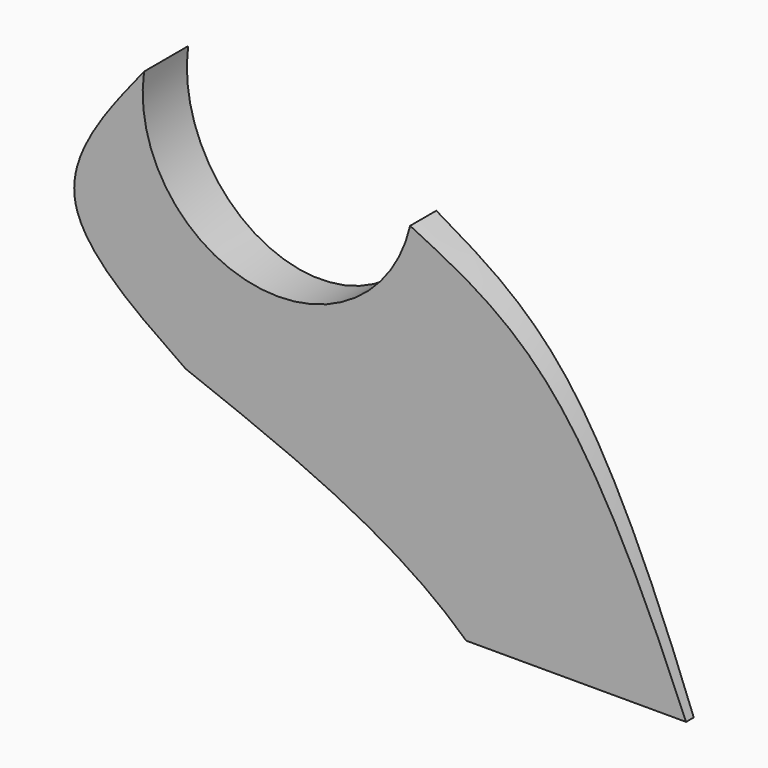
from build123d import *

# Parameters (mm, degrees)
F2_DEPTH = 25.7279276848
F3_DEPTH = 102.7941810931


# Not quite as in the source:
# - a feature names something its author has since deleted; it is built from what else it names


with BuildPart() as f2:
    # F0 (on Front) → F2 (new body, through all)
    with BuildSketch(Plane.XZ):
        with BuildLine():
            ThreePointArc((7.538071066, 90.012077608), (-33.0999025849, 63.2971569556), (-61.4758778659, 102.7931809931))
            add(Edge.make_bspline(
                [(-50.6802275777, 38.4073108435), (-64.2301253741, 47.6853026647), (-91.0055411856, 66.0246371681), (-71.2591028819, 90.6346541889), (-61.4758778659, 102.7931809931)],
                knots=[0, 0, 0, 0, 0.5057307672, 1, 1, 1, 1], degree=3))
            add(Edge.make_bspline(
                [(62.097594142, -64.207687974), (51.1832226367, -40.5716055165), (28.887804967, 7.7111846278), (-23.7900094582, 28.033475615), (-50.6802275777, 38.4073108435)],
                knots=[0, 0, 0, 0, 0.4895343419, 1, 1, 1, 1], degree=3))
            Line((62.097594142, -64.207687974), (96.4130014181, -43.6846762896))
            add(Edge.make_bspline(
                [(96.4130014181, -43.6846762896), (79.9973481318, -1.0988161117), (53.4561883249, 67.712624491), (20.2239489646, 83.857797394), (7.538071066, 90.012077608)],
                knots=[0, 0, 0, 0, 0.6187491541, 1, 1, 1, 1], degree=3))
        make_face()
    extrude(amount=F2_DEPTH)


with BuildPart() as f3:
    # F1 (on Top) → F3 (new body, through all)
    with BuildSketch(Plane.XY):
        Polygon((108.6692065001, -25.7279276848), (-108.6692065001, -7.4702873826), (-108.6692065001, -25.7279276848), align=None)
    extrude(amount=F3_DEPTH)

    # F4: intersect F2
    add(f2.part, mode=Mode.INTERSECT)


solid = f3.part
